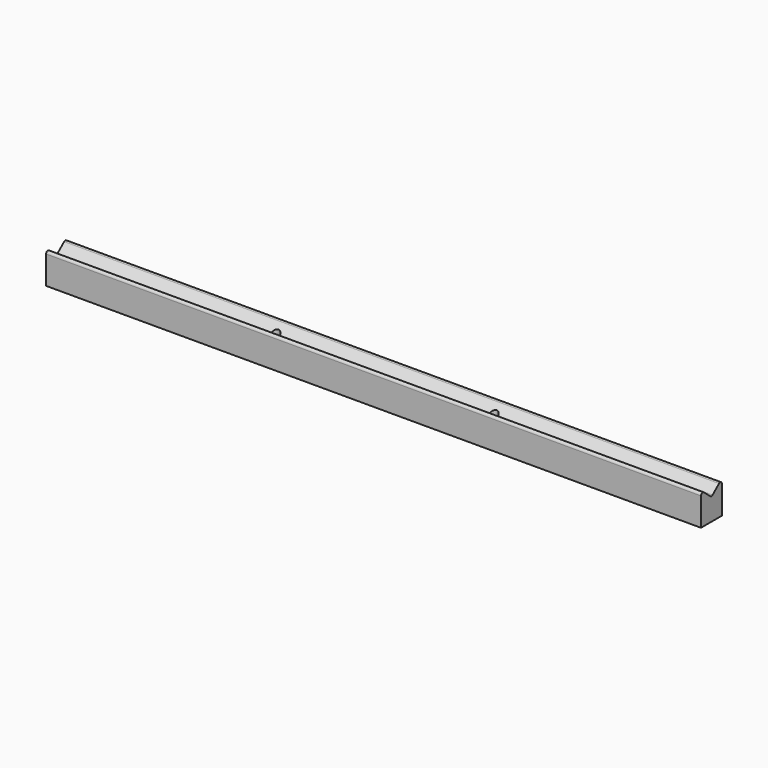
from build123d import *

# Parameters (mm, degrees)
F0_W         = 300
F0_H         = 12
F0_R         = 2
F1_DEPTH     = 15
F3_DEPTH     = 300.001
F4_T4_DEPTH  = 100.0833333333
F4_S5_R      = 2
F4_T6_DEPTH  = 52
F4_T10_DEPTH = 100.1666666667
F4_S11_R     = 2
F4_T12_DEPTH = 52
F4_S13_R     = 2
F4_T14_DEPTH = 52
F4_T18_DEPTH = 100.0833333333
F4_S19_R     = 2
F4_T20_DEPTH = 52
F4_T21_DEPTH = 310.6752080633


# Not quite as in the source:
# - a fillet or chamfer that OpenCascade refuses, or shapes differently, is made with other operations: its cross-section is extruded or revolved along the edge and cut away or added


with BuildPart() as f1:
    # F0 (on Top) → F1 (new body)
    with BuildSketch(Plane.XY):
        Rectangle(F0_W, F0_H)
        with Locations((-50, 0)):
            Circle(F0_R, mode=Mode.SUBTRACT)
        with Locations((50, 0)):
            Circle(F0_R, mode=Mode.SUBTRACT)
    extrude(amount=F1_DEPTH)

    # F2 (on face) → F3 (cut, through all)
    with BuildSketch(Plane.YZ.offset(150)):
        Polygon((6, 15), (-6, 15), (0, 10), align=None)
    extrude(amount=-F3_DEPTH, mode=Mode.SUBTRACT)

    # F4: fillet of radius 1 on 5 edges, made by hand


with BuildPart() as f4_tool2:
    # F4_s3 → F4_t4 (new body)
    with BuildSketch(Plane.YZ.offset(150)):
        with BuildLine():
            ThreePointArc((-0.6401843997, 10.5334869997), (0, 10.3017082793), (0.6401843997, 10.5334869997))
            Line((0.6401843997, 10.5334869997), (0, 10))
            Line((0, 10), (-0.6401843997, 10.5334869997))
        make_face()
    extrude(amount=-F4_T4_DEPTH)

    # F4_s5 → F4_t6 (cut, symmetric)
    with BuildSketch(Plane.XY.offset(10.3)):
        with Locations((50, 0)):
            Circle(F4_S5_R)
    extrude(amount=F4_T6_DEPTH, both=True, mode=Mode.SUBTRACT)


with BuildPart() as f1_1:
    add(f1.part)

    # F4_t1: union F4_tool2
    add(f4_tool2.part)


with BuildPart() as f4_tool8:
    # F4_s9 → F4_t10 (new body)
    with BuildSketch(Plane.YZ.offset(50.0833333333)):
        with BuildLine():
            ThreePointArc((-0.6401843997, 10.5334869997), (0, 10.3017082793), (0.6401843997, 10.5334869997))
            Line((0.6401843997, 10.5334869997), (0, 10))
            Line((0, 10), (-0.6401843997, 10.5334869997))
        make_face()
    extrude(amount=-F4_T10_DEPTH)

    # F4_s11 → F4_t12 (cut, symmetric)
    with BuildSketch(Plane.XY.offset(10.3)):
        with Locations((50, 0)):
            Circle(F4_S11_R)
    extrude(amount=F4_T12_DEPTH, both=True, mode=Mode.SUBTRACT)

    # F4_s13 → F4_t14 (cut, symmetric)
    with BuildSketch(Plane.XY.offset(10.3)):
        with Locations((-50, 0)):
            Circle(F4_S13_R)
    extrude(amount=F4_T14_DEPTH, both=True, mode=Mode.SUBTRACT)


with BuildPart() as f1_2:
    add(f1_1.part)

    # F4_t7: union F4_tool8
    add(f4_tool8.part)


with BuildPart() as f4_tool16:
    # F4_s17 → F4_t18 (new body)
    with BuildSketch(Plane.YZ.offset(-49.9166666667)):
        with BuildLine():
            ThreePointArc((-0.6401843997, 10.5334869997), (0, 10.3017082793), (0.6401843997, 10.5334869997))
            Line((0.6401843997, 10.5334869997), (0, 10))
            Line((0, 10), (-0.6401843997, 10.5334869997))
        make_face()
    extrude(amount=-F4_T18_DEPTH)

    # F4_s19 → F4_t20 (cut, symmetric)
    with BuildSketch(Plane.XY.offset(10.3)):
        with Locations((-50, 0)):
            Circle(F4_S19_R)
    extrude(amount=F4_T20_DEPTH, both=True, mode=Mode.SUBTRACT)


with BuildPart() as f1_3:
    add(f1_2.part)

    # F4_t15: union F4_tool16
    add(f4_tool16.part)

    # F4_s22 → F4_t21 (cut)
    with BuildSketch(Plane.YZ.offset(-155.3376040316)):
        with BuildLine():
            ThreePointArc((-6, 12.8649583873), (-5.4241553962, 13.7705478086), (-4.3598156003, 13.6331796669))
            Line((-4.3598156003, 13.6331796669), (-6, 15))
            Line((-6, 15), (-6, 12.8649583873))
        make_face()
        with BuildLine():
            ThreePointArc((4.3598156003, 13.6331796669), (5.4241553962, 13.7705478086), (6, 12.8649583873))
            Line((6, 12.8649583873), (6, 15))
            Line((6, 15), (4.3598156003, 13.6331796669))
        make_face()
    extrude(amount=F4_T21_DEPTH, mode=Mode.SUBTRACT)


solid = f1_3.part
